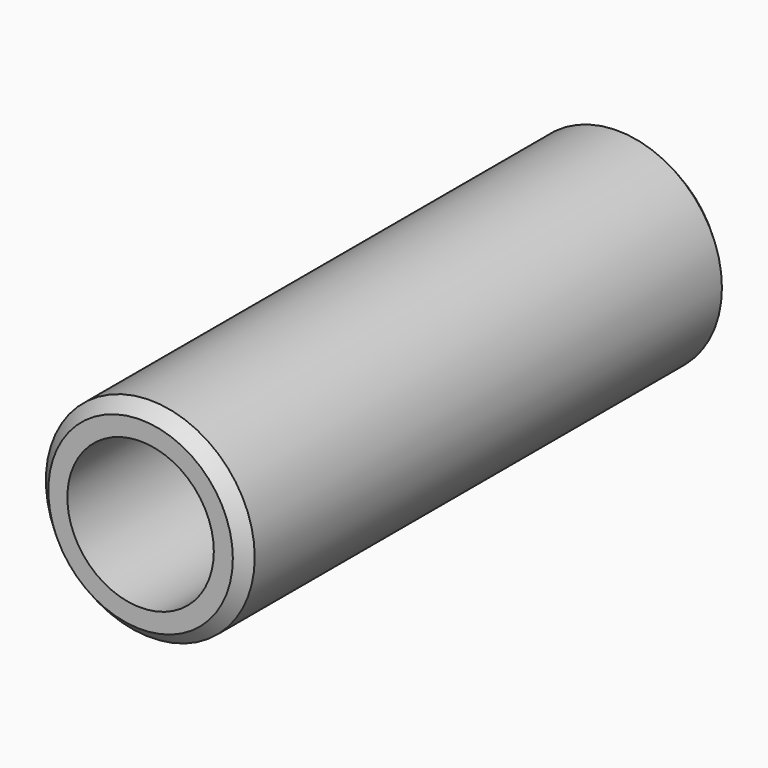
from build123d import *

# Parameters (mm, degrees)
F0_R     = 43.605966959
F0_R_2   = 30.5874681623
F1_DEPTH = 254
F4_SIZE  = 5.08


# Not quite as in the source:
# - the program builds the solid bodies; features that only make, move or delete a surface that nothing else refers to are left out


with BuildPart() as f1:
    # F0 (on Front) → F1 (new body)
    with BuildSketch(Plane.XZ):
        Circle(F0_R)
        Circle(F0_R_2, mode=Mode.SUBTRACT)
    extrude(amount=F1_DEPTH)

    # F4
    f4_edges = [f1.edges().sort_by_distance(p)[0] for p in [
        (43.605967, -127, 0),
        (-43.605967, 0, 0),
        (-43.605967, -254, 0),
    ]]
    chamfer(f4_edges, length=F4_SIZE)


solid = f1.part
